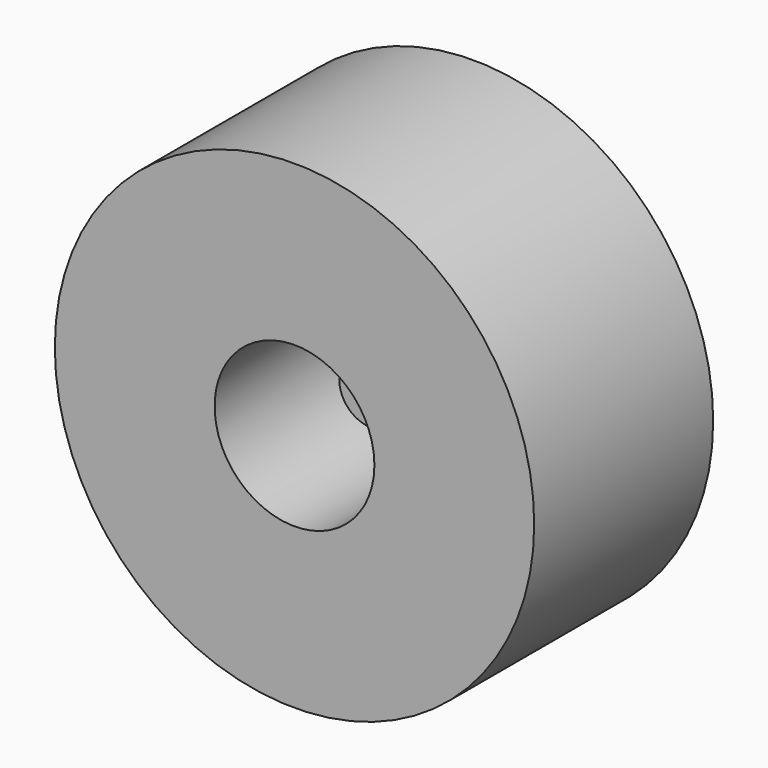
from build123d import *

# Parameters (mm, degrees)
F0_R      = 19.05
F1_DEPTH  = 17.78
F4_R      = 6.35
F4_R_2    = 2.5388917956
F5_DEPTH  = 12.7
F2_R      = 2.5388917956
F2_R_2    = 2.4229582781
F6_DEPTH  = 7.62
F8_R      = 1.2674888325
F9_DEPTH  = 2.54
F10_DEPTH = 25.4
F11_R     = 2.5702523623
F3_R      = 2.519460743
F12_DEPTH = 12.7


# Not quite as in the source:
# - a feature of the source that left no trace in its solid (it failed there, or was rolled back) is left out


with BuildPart() as f1:
    # F0 (on Front) → F1 (new body)
    with BuildSketch(Plane.XZ):
        Circle(F0_R)
    extrude(amount=F1_DEPTH)

    # F4 (on face) → F5 (cut)
    with BuildSketch(Plane.XZ.offset(17.78)):
        Circle(F4_R)
        Circle(F4_R_2, mode=Mode.SUBTRACT)
    extrude(amount=-F5_DEPTH, mode=Mode.SUBTRACT)

    # F2 (on face) → F6 (cut)
    with BuildSketch(Plane.XZ.offset(17.78)):
        Circle(F2_R)
        Circle(F2_R_2, mode=Mode.SUBTRACT)
        Circle(F2_R_2)
    extrude(amount=-F6_DEPTH, mode=Mode.SUBTRACT)

    # F8 (on face) → F9 (cut)
    with BuildSketch(Plane.XZ.offset(5.08)):
        with Locations((-4.2412145995, 0)):
            Circle(F8_R)
        with Locations((-2.9989916037, 2.9989916037)):
            Circle(F8_R)
        with Locations((0, 4.2412145995)):
            Circle(F8_R)
        with Locations((2.9989916037, 2.9989916037)):
            Circle(F8_R)
        with Locations((4.2412145995, 0)):
            Circle(F8_R)
        with Locations((2.9989916037, -2.9989916037)):
            Circle(F8_R)
        with Locations((0, -4.2412145995)):
            Circle(F8_R)
        with Locations((-2.9989916037, -2.9989916037)):
            Circle(F8_R)
    extrude(amount=-F9_DEPTH, mode=Mode.SUBTRACT)

    # F10 (cut): faces of the model
    f10_faces = [f1.faces().sort_by_distance(p)[0] for p in [
        (-2.9989916037, -2.54, 2.9989916037),
        (-4.2412145995, -2.54, 0),
        (-2.9989916037, -2.54, -2.9989916037),
        (0, -2.54, -4.2412145995),
        (2.9989916037, -2.54, -2.9989916037),
        (4.2412145995, -2.54, 0),
        (2.9989916037, -2.54, 2.9989916037),
        (0, -2.54, 4.2412145995),
    ]]
    extrude(f10_faces, amount=-F10_DEPTH, mode=Mode.SUBTRACT)

    # F11 (on face) + F3 (on face) → F12 (join)
    with BuildSketch(Plane(origin=(0, 0, 0), x_dir=(-1, 0, 0), z_dir=(0, 1, 0))):
        Circle(F11_R)
    with BuildSketch(Plane(origin=(0, 0, 0), x_dir=(-1, 0, 0), z_dir=(0, 1, 0))):
        Circle(F3_R)
    extrude(amount=F12_DEPTH)


solid = f1.part
